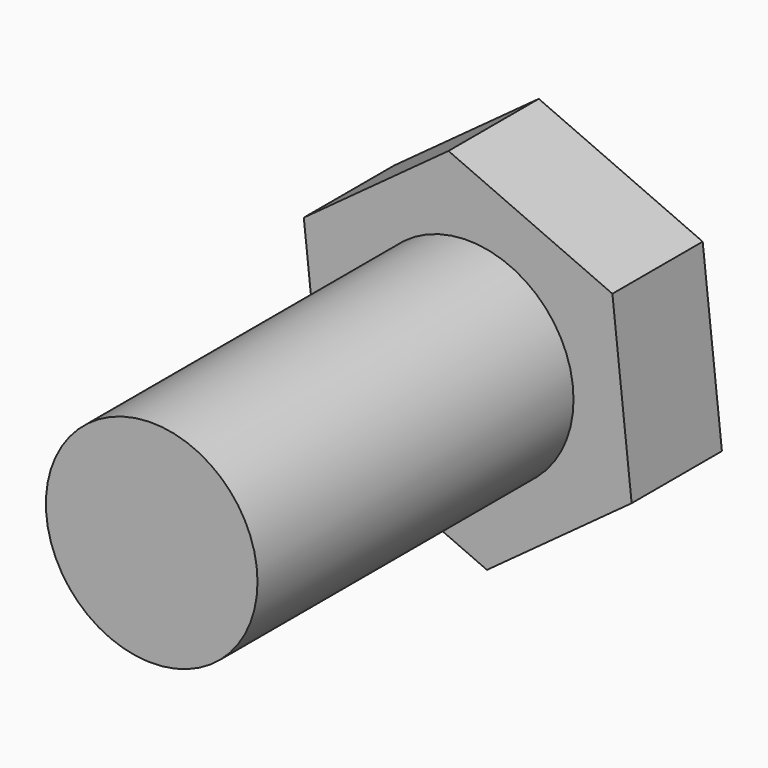
from build123d import *

# Parameters (mm, degrees)
F1_DEPTH = 4
F2_R     = 3.75
F3_DEPTH = 14


# Not quite as in the source:
# - a feature names something its author has since deleted; it is built from what else it names


with BuildPart() as f1:
    # F0 (on Front) → F1 (new body)
    with BuildSketch(Plane.XZ):
        Polygon((0.6816548843, -6.3141650241), (5.8090547568, -2.5667520656), (5.1273998724, 3.7474129585), (-0.6816548843, 6.3141650241), (-5.8090547568, 2.5667520656), (-5.1273998724, -3.7474129585), align=None)
    extrude(amount=F1_DEPTH)

    # F2 (on face) → F3 (join)
    with BuildSketch(Plane.XZ.offset(4)):
        Circle(F2_R)
    extrude(amount=F3_DEPTH)


solid = f1.part
